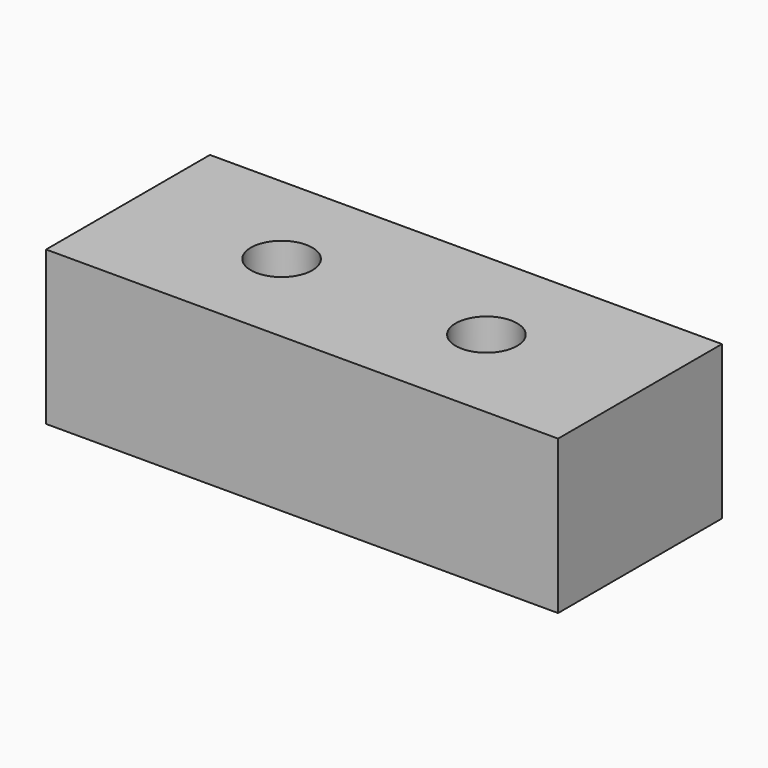
from build123d import *

# Parameters (mm, degrees)
F0_W     = 63.5
F0_H     = 19.05
F1_DEPTH = 12.7
F2_R     = 3.81
F3_DEPTH = 12.7


# Not quite as in the source:
# - a feature names something its author has since deleted; it is built from what else it names


with BuildPart() as f1:
    # F0 (on Front) → F1 (new body, symmetric)
    with BuildSketch(Plane.XZ):
        with Locations((31.75, -9.525)):
            Rectangle(F0_W, F0_H)
    extrude(amount=F1_DEPTH, both=True)

    # F2 (on face) → F3 (cut)
    with BuildSketch(Plane.XY):
        with Locations((44.45, 0)):
            Circle(F2_R)
        with Locations((19.05, 0)):
            Circle(F2_R)
    extrude(amount=-F3_DEPTH, mode=Mode.SUBTRACT)


solid = f1.part
